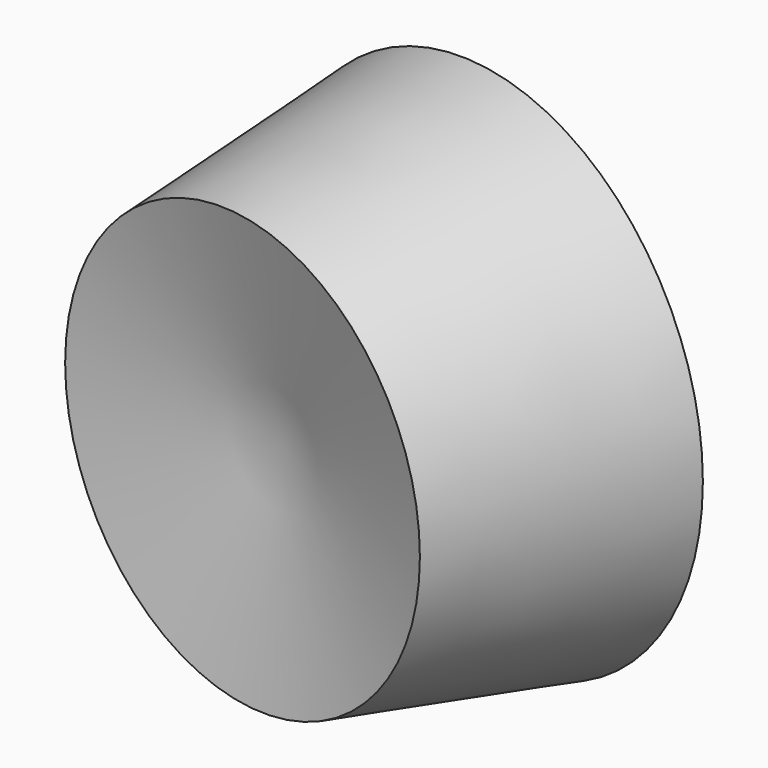
from build123d import *


with BuildPart() as f1:
    # F0 (on Top) → F1 (revolve)
    with BuildSketch(Plane.XY):
        Polygon((-0.20721069, 0.2180140772), (-46.4914007533, 55.0688933581), (-47.8657117786, -44.9998579924), align=None)
        Polygon((37.9484690832, -44.9998579924), (-0.20721069, 0.2180140772), (-47.8657117786, -44.9998579924), align=None)
        Polygon((57.6042379755, 55.0688933581), (-0.20721069, 0.2180140772), (37.9484690832, -44.9998579924), align=None)
    revolve(axis=Axis((47.7763535294, 5.0345176828, 0), (-0.1927397054, -0.9812499202, 0)))


solid = f1.part
